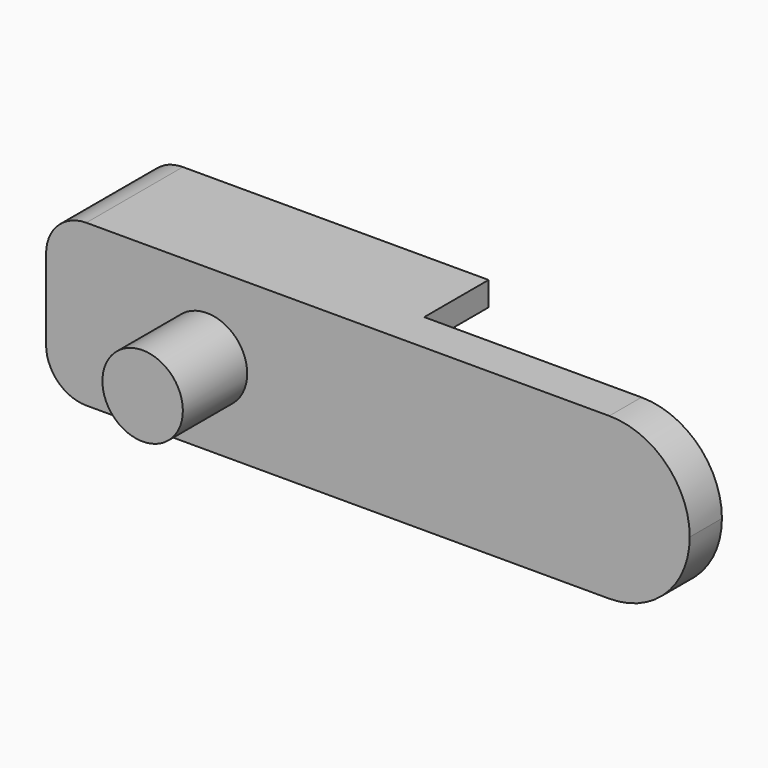
from build123d import *

# Parameters (mm, degrees)
F0_W     = 50.8
F0_H     = 12.7
F1_DEPTH = 3.175
F2_R     = 3.175
F3_DEPTH = 6.35
F5_DEPTH = 6.35
F6_R     = 6.34999
F7_R     = 3.175


# Not quite as in the source:
# - a fillet or chamfer is up to 0.001 mm smaller than in the source, because OpenCascade refuses the exact size


with BuildPart() as f1:
    # F0 (on Front) → F1 (new body)
    with BuildSketch(Plane.XZ):
        with Locations((15.0143924374, -1.4320164919)):
            Rectangle(F0_W, F0_H)
    extrude(amount=F1_DEPTH)

    # F2 (on face) → F3 (join)
    with BuildSketch(Plane.XZ.offset(3.175)):
        with Locations((2.3143924374, -1.4320164919)):
            Circle(F2_R)
    extrude(amount=F3_DEPTH)

    # F4 (on face) → F5 (join)
    with BuildSketch(Plane(origin=(0, 0, 0), x_dir=(-1, 0, 0), z_dir=(0, 1, 0))):
        Polygon((8.4806075626, 3.0129835081), (8.4806075626, -5.8770164919), (-16.9193924374, -5.8770164919), (-16.9193924374, -7.7820164919), (10.3856075626, -7.7820164919), (10.3856075626, 4.9179835081), (-16.9193924374, 4.9179835081), (-16.9193924374, 3.0129835081), align=None)
    extrude(amount=F5_DEPTH)

    # F6 (radius 6.35 in the source; OpenCascade refuses exactly that, so slightly less here)
    f6_edges = [f1.edges().sort_by_distance(p)[0] for p in [
        (40.414392, -1.5875, 4.917984),
        (40.414392, -1.5875, -7.782016),
    ]]
    fillet(f6_edges, radius=F6_R)

    # F7
    f7_edges = [f1.edges().sort_by_distance(p)[0] for p in [
        (-8.480608, 3.175, 3.012984),
        (-8.480608, 3.175, -5.877016),
        (-10.385608, 1.5875, 4.917984),
        (-10.385608, 1.5875, -7.782016),
    ]]
    fillet(f7_edges, radius=F7_R)


solid = f1.part
